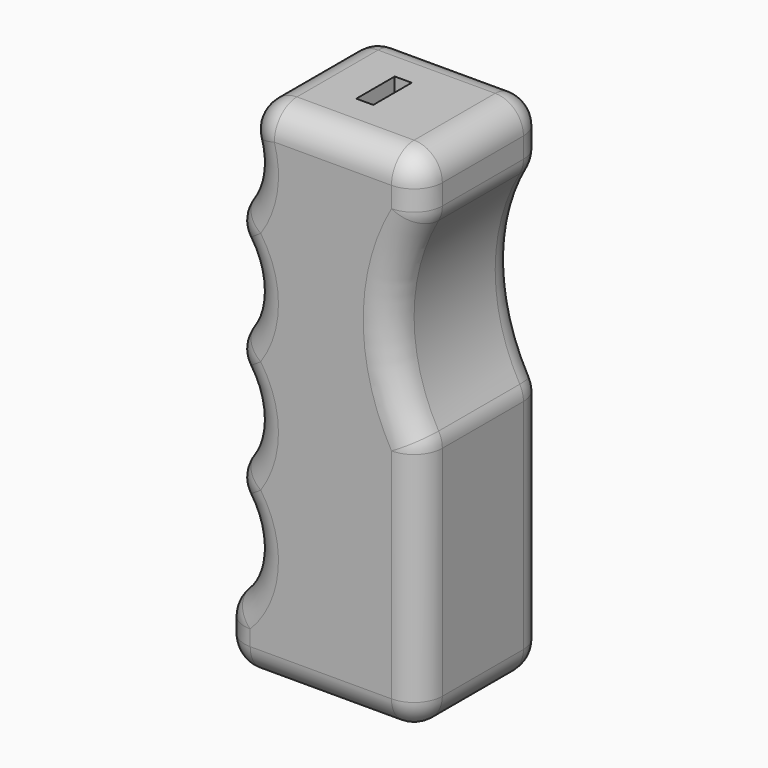
from build123d import *

# Parameters (mm, degrees)
F0_W     = 35
F0_H     = 90
F1_DEPTH = 27.94
F3_DEPTH = 27.941
F4_W     = 3
F4_H     = 8.5
F5_DEPTH = 30
F6_R     = 5


with BuildPart() as f1:
    # F0 (on Front) → F1 (new body)
    with BuildSketch(Plane.XZ):
        with Locations((17.5, 45)):
            Rectangle(F0_W, F0_H)
    extrude(amount=F1_DEPTH)

    # F2 (on face) → F3 (cut, through all)
    with BuildSketch(Plane.XZ.offset(27.94)):
        with BuildLine():
            Line((35, 45), (35, 80))
            ThreePointArc((35, 80), (30, 62.5), (35, 45))
        make_face()
        with BuildLine():
            ThreePointArc((0, 70), (5, 80), (0, 90))
            Line((0, 90), (0, 70))
        make_face()
        with BuildLine():
            ThreePointArc((0, 50), (5, 60), (0, 70))
            Line((0, 70), (0, 50))
        make_face()
        with BuildLine():
            ThreePointArc((0, 30), (5, 40), (0, 50))
            Line((0, 50), (0, 30))
        make_face()
        with BuildLine():
            Line((0, 30), (0, 10))
            ThreePointArc((0, 10), (5, 20), (0, 30))
        make_face()
    extrude(amount=-F3_DEPTH, mode=Mode.SUBTRACT)

    # F4 (on face) → F5 (cut)
    with BuildSketch(Plane.XY.offset(90)):
        with Locations((17.5, -13.97)):
            Rectangle(F4_W, F4_H)
    extrude(amount=-F5_DEPTH, mode=Mode.SUBTRACT)

    # F6
    f6_edges = [f1.edges().sort_by_distance(p)[0] for p in [
        (5, -27.94, 60),
        (0, -13.97, 70),
        (5, 0, 60),
        (0, -13.97, 50),
        (5, -27.94, 80),
        (0, -13.97, 90),
        (5, 0, 80),
        (5, 0, 40),
        (5, -27.94, 40),
        (0, 0, 5),
        (0, -13.97, 0),
        (0, -27.94, 5),
        (0, -13.97, 10),
        (35, -13.97, 0),
        (17.5, 0, 0),
        (17.5, -27.94, 0),
        (35, 0, 22.5),
        (35, -13.97, 45),
        (35, -27.94, 22.5),
        (30, -27.94, 62.5),
        (30, 0, 62.5),
        (35, -13.97, 80),
        (35, 0, 85),
        (35, -13.97, 90),
        (35, -27.94, 85),
        (17.5, 0, 90),
        (17.5, -27.94, 90),
        (5, -27.94, 20),
        (5, 0, 20),
        (0, -13.97, 30),
    ]]
    fillet(f6_edges, radius=F6_R)


solid = f1.part
